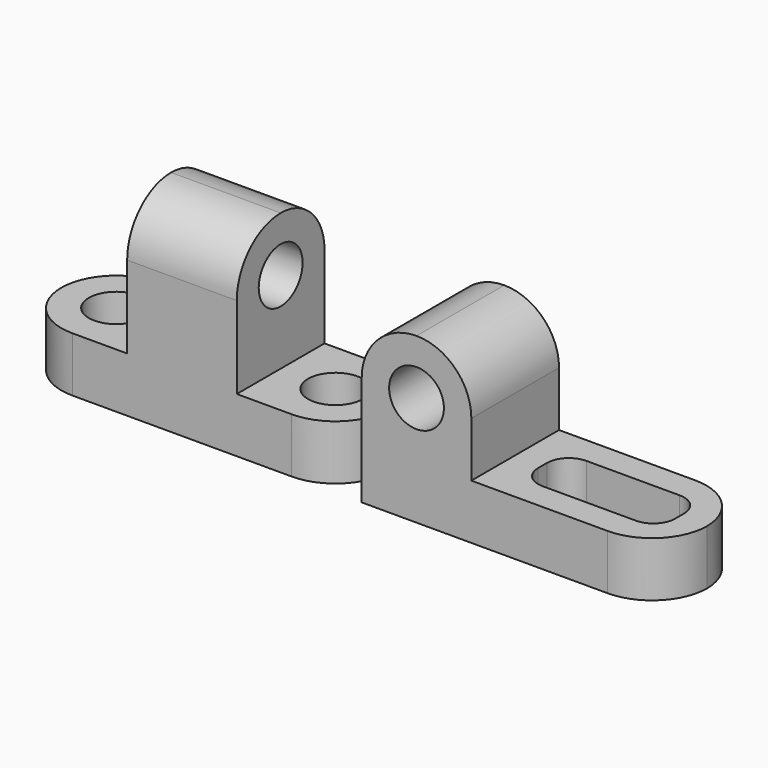
from build123d import *

# Parameters (mm, degrees)
F0_W         = 69.85
F0_H         = 25.4
F1_DEPTH     = 12.7
F2_W         = 25.4
F2_H         = 25.4
F3_DEPTH     = 25.4
F5_D         = 12.7
F6_W         = 31.75
F6_H         = 12.7
F7_DEPTH     = 12.7
F9_DEPTH     = 25.4
F10_DEPTH    = 25.4
F11_R        = 5.08
F12_T1_DEPTH = 77.0870757085
F13_W        = 76.2
F13_H        = 25.4
F14_DEPTH    = 12.7
F15_W        = 25.4
F15_H        = 25.4
F16_DEPTH    = 31.75
F17_R        = 6.35
F18_DEPTH    = 12.7
F19_R        = 6.35
F20_DEPTH    = 12.7
F21_R        = 6.35
F22_DEPTH    = 25.4


# Not quite as in the source:
# - a fillet or chamfer that OpenCascade refuses, or shapes differently, is made with other operations: its cross-section is extruded or revolved along the edge and cut away or added


with BuildPart() as f1:
    # F0 (on Top) → F1 (new body)
    with BuildSketch(Plane.XY):
        with Locations((34.925, 12.7)):
            Rectangle(F0_W, F0_H)
    extrude(amount=F1_DEPTH)

    # F2 (on face) → F3 (join)
    with BuildSketch(Plane.XY.offset(12.7)):
        with Locations((12.7, 12.7)):
            Rectangle(F2_W, F2_H)
    extrude(amount=F3_DEPTH)

    # F5 (through all)
    with Locations(Plane.XZ):
        with Locations((12.7, 25.4)):
            Hole(F5_D / 2)

    # F6 (on face) → F7 (cut)
    with BuildSketch(Plane.XY.offset(12.7)):
        with Locations((47.625, 12.7)):
            Rectangle(F6_W, F6_H)
    extrude(amount=-F7_DEPTH, mode=Mode.SUBTRACT)

    # F8 (on face) → F9 (cut)
    with BuildSketch(Plane.XZ):
        with BuildLine():
            ThreePointArc((0, 25.4), (3.7197438789, 34.3802561211), (12.7, 38.1))
            Line((12.7, 38.1), (0, 38.1))
            Line((0, 38.1), (0, 25.4))
        make_face()
    extrude(amount=-F9_DEPTH, mode=Mode.SUBTRACT)

    # F8 (on face) → F10 (cut)
    with BuildSketch(Plane.XZ):
        with BuildLine():
            ThreePointArc((12.7, 38.1), (21.6802561211, 34.3802561211), (25.4, 25.4))
            Line((25.4, 25.4), (25.4, 38.1))
            Line((25.4, 38.1), (12.7, 38.1))
        make_face()
    extrude(amount=-F10_DEPTH, mode=Mode.SUBTRACT)

    # F11
    f11_edges = [f1.edges().sort_by_distance(p)[0] for p in [
        (31.75, 19.05, 6.35),
        (31.75, 6.35, 6.35),
        (63.5, 19.05, 6.35),
        (63.5, 6.35, 6.35),
    ]]
    fillet(f11_edges, radius=F11_R)

    # F12: fillet of radius 12.8774151417 on 2 edges, made by hand

    # F12_s2 → F12_t1 (cut)
    with BuildSketch(Plane.XY.offset(-32.1935378542)):
        with BuildLine():
            ThreePointArc((56.9725848583, 25.4), (66.0782924292, 21.6282924292), (69.85, 12.5225848583))
            Line((69.85, 12.5225848583), (69.85, 25.4))
            Line((69.85, 25.4), (56.9725848583, 25.4))
        make_face()
        with BuildLine():
            ThreePointArc((69.85, 12.8774151417), (66.0782924292, 3.7717075708), (56.9725848583, 0))
            Line((56.9725848583, 0), (69.85, 0))
            Line((69.85, 0), (69.85, 12.8774151417))
        make_face()
    extrude(amount=F12_T1_DEPTH, mode=Mode.SUBTRACT)


with BuildPart() as f14:
    # F13 (on Top) → F14 (new body)
    with BuildSketch(Plane.XY):
        with Locations((-41.638404093, 12.7)):
            Rectangle(F13_W, F13_H)
    extrude(amount=F14_DEPTH)

    # F15 (on face) → F16 (join)
    with BuildSketch(Plane.XY.offset(12.7)):
        with Locations((-41.638404093, 12.7)):
            Rectangle(F15_W, F15_H)
    extrude(amount=F16_DEPTH)

    # F17 (on face) → F18 (cut)
    with BuildSketch(Plane.XY.offset(12.7)):
        with Locations((-16.238404093, 12.7)):
            Circle(F17_R)
        with BuildLine():
            ThreePointArc((-16.238404093, 25.4), (-7.2581479719, 21.6802561211), (-3.538404093, 12.7))
            Line((-3.538404093, 12.7), (-3.538404093, 25.4))
            Line((-3.538404093, 25.4), (-16.238404093, 25.4))
        make_face()
        with BuildLine():
            ThreePointArc((-3.538404093, 12.7), (-7.2581479719, 3.7197438789), (-16.238404093, 0))
            Line((-16.238404093, 0), (-3.538404093, 0))
            Line((-3.538404093, 0), (-3.538404093, 12.7))
        make_face()
    extrude(amount=-F18_DEPTH, mode=Mode.SUBTRACT)

    # F19 (on face) → F20 (cut)
    with BuildSketch(Plane.XY.offset(12.7)):
        with Locations((-67.038404093, 12.7)):
            Circle(F19_R)
        with BuildLine():
            ThreePointArc((-79.738404093, 12.7), (-76.0186602141, 21.6802561211), (-67.038404093, 25.4))
            Line((-67.038404093, 25.4), (-79.738404093, 25.4))
            Line((-79.738404093, 25.4), (-79.738404093, 12.7))
        make_face()
        with BuildLine():
            ThreePointArc((-67.038404093, 0), (-76.0186602141, 3.7197438789), (-79.738404093, 12.7))
            Line((-79.738404093, 12.7), (-79.738404093, 0))
            Line((-79.738404093, 0), (-67.038404093, 0))
        make_face()
    extrude(amount=-F20_DEPTH, mode=Mode.SUBTRACT)

    # F21 (on face) → F22 (cut)
    with BuildSketch(Plane(origin=(-54.338404093, 0, 0), x_dir=(0, -1, 0), z_dir=(-1, 0, 0))):
        with Locations((-12.7, 31.75)):
            Circle(F21_R)
        with BuildLine():
            ThreePointArc((-25.4, 31.75), (-21.6802561211, 40.7302561211), (-12.7, 44.45))
            Line((-12.7, 44.45), (-25.4, 44.45))
            Line((-25.4, 44.45), (-25.4, 31.75))
        make_face()
        with BuildLine():
            ThreePointArc((-12.7, 44.45), (-3.7197438789, 40.7302561211), (0, 31.75))
            Line((0, 31.75), (0, 44.45))
            Line((0, 44.45), (-12.7, 44.45))
        make_face()
    extrude(amount=-F22_DEPTH, mode=Mode.SUBTRACT)


solid = Compound([f1.part, f14.part])
